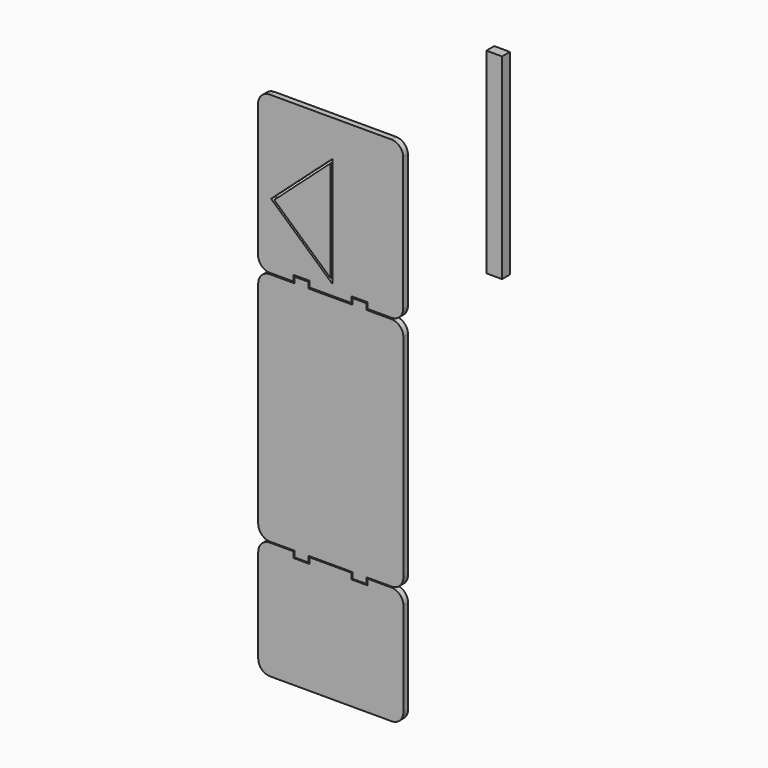
from build123d import *

# Parameters (mm, degrees)
F1_DEPTH = 15
F2_DEPTH = 15
F0_W     = 40
F0_H     = 500
F3_DEPTH = 25


# Not quite as in the source:
# - a feature names something its author has since deleted; it is built from what else it names


with BuildPart() as f1:
    # F0 (on Front) → F1 (new body)
    with BuildSketch(Plane.XZ):
        with BuildLine():
            Line((157.9930828999, 251.0488363948), (-152.0069171001, 251.0488363948))
            ThreePointArc((-152.0069171001, 251.0488363948), (-173.2201205357, 242.2620398304), (-182.0069171001, 221.0488363948))
            Line((-182.0069171001, 221.0488363948), (-182.0069171001, -118.9511636052))
            ThreePointArc((-182.0069171001, -118.9511636052), (-173.2201205357, -140.1643670408), (-152.0069171001, -148.9511636052))
            Line((-152.0069171001, -148.9511636052), (-91.4793238044, -148.9511636052))
            Line((-91.4793238044, -148.9511636052), (-91.4793238044, -133.9511636052))
            Line((-91.4793238044, -133.9511636052), (-51.4793238044, -133.9511636052))
            Line((-51.4793238044, -133.9511636052), (-51.4793238044, -148.9511636052))
            Line((-51.4793238044, -148.9511636052), (56.4180724323, -148.9511636052))
            Line((56.4180724323, -148.9511636052), (56.4180724323, -133.9511636052))
            Line((56.4180724323, -133.9511636052), (96.4180724323, -133.9511636052))
            Line((96.4180724323, -133.9511636052), (96.4180724323, -148.9511636052))
            Line((96.4180724323, -148.9511636052), (157.9930828999, -148.9511636052))
            ThreePointArc((157.9930828999, -148.9511636052), (179.2062863355, -140.1643670408), (187.9930828999, -118.9511636052))
            Line((187.9930828999, -118.9511636052), (187.9930828999, 221.0488363948))
            ThreePointArc((187.9930828999, 221.0488363948), (179.2062863355, 242.2620398304), (157.9930828999, 251.0488363948))
        make_face()
        Polygon((8.2889962941, 159.2487096786), (8.2889962941, -122.7074861526), (-148.9303992233, 18.270611763), align=None, mode=Mode.SUBTRACT)
    extrude(amount=F1_DEPTH)


with BuildPart() as f2:
    # F0 (on Front) → F2 (new body)
    with BuildSketch(Plane.XZ):
        with BuildLine():
            Line((-89.0557542443, -152.287649894), (-151.6510576755, -152.287649894))
            ThreePointArc((-151.6510576755, -152.287649894), (-172.8642611111, -161.0744464584), (-181.6510576755, -182.287649894))
            Line((-181.6510576755, -182.287649894), (-181.6510576755, -722.287649894))
            ThreePointArc((-181.6510576755, -722.287649894), (-172.8642611111, -743.5008533296), (-151.6510576755, -752.287649894))
            Line((-151.6510576755, -752.287649894), (-88.8991951942, -752.287649894))
            Line((-88.8991951942, -752.287649894), (-88.8991951942, -767.287649894))
            Line((-88.8991951942, -767.287649894), (-53.8991951942, -767.287649894))
            Line((-53.8991951942, -767.287649894), (-53.8991951942, -752.287649894))
            Line((-53.8991951942, -752.287649894), (59.3375265598, -752.287649894))
            Line((59.3375265598, -752.287649894), (59.3375265598, -767.287649894))
            Line((59.3375265598, -767.287649894), (94.3375265598, -767.287649894))
            Line((94.3375265598, -767.287649894), (94.3375265598, -752.287649894))
            Line((94.3375265598, -752.287649894), (158.3489423245, -752.287649894))
            ThreePointArc((158.3489423245, -752.287649894), (179.5621457601, -743.5008533296), (188.3489423245, -722.287649894))
            Line((188.3489423245, -722.287649894), (188.3489423245, -182.287649894))
            ThreePointArc((188.3489423245, -182.287649894), (179.5621457601, -161.0744464584), (158.3489423245, -152.287649894))
            Line((158.3489423245, -152.287649894), (94.114292264, -152.287649894))
            Line((94.114292264, -152.287649894), (94.114292264, -137.287649894))
            Line((94.114292264, -137.287649894), (59.114292264, -137.287649894))
            Line((59.114292264, -137.287649894), (59.114292264, -152.287649894))
            Line((59.114292264, -152.287649894), (-54.0557542443, -152.287649894))
            Line((-54.0557542443, -152.287649894), (-54.0557542443, -137.287649894))
            Line((-54.0557542443, -137.287649894), (-89.0557542443, -137.287649894))
            Line((-89.0557542443, -137.287649894), (-89.0557542443, -152.287649894))
        make_face()
    extrude(amount=F2_DEPTH)


with BuildPart() as f2b:
    # F0 (on Front) → F2, piece 2 (new body)
    with BuildSketch(Plane.XZ):
        with BuildLine():
            Line((-91.2640253641, -754.7138333321), (-151.6000044346, -754.7138333321))
            ThreePointArc((-151.6000044346, -754.7138333321), (-172.8132078702, -763.5006298965), (-181.6000044346, -784.7138333321))
            Line((-181.6000044346, -784.7138333321), (-181.6000044346, -1024.7138333321))
            ThreePointArc((-181.6000044346, -1024.7138333321), (-172.8132078702, -1045.9270367677), (-151.6000044346, -1054.7138333321))
            Line((-151.6000044346, -1054.7138333321), (-91.3764173724, -1054.7138333321))
            Line((-91.3764173724, -1054.7138333321), (56.5209788643, -1054.7138333321))
            Line((56.5209788643, -1054.7138333321), (158.3999955654, -1054.7138333321))
            ThreePointArc((158.3999955654, -1054.7138333321), (179.613199001, -1045.9270367677), (188.3999955654, -1024.7138333321))
            Line((188.3999955654, -1024.7138333321), (188.3999955654, -784.7138333321))
            ThreePointArc((188.3999955654, -784.7138333321), (179.613199001, -763.5006298965), (158.3999955654, -754.7138333321))
            Line((158.3999955654, -754.7138333321), (96.4699256234, -754.7138333321))
            Line((96.4699256234, -754.7138333321), (96.4699256234, -769.7138333321))
            Line((96.4699256234, -769.7138333321), (56.4699256234, -769.7138333321))
            Line((56.4699256234, -769.7138333321), (56.4699256234, -754.7138333321))
            Line((56.4699256234, -754.7138333321), (-51.2640253641, -754.7138333321))
            Line((-51.2640253641, -754.7138333321), (-51.2640253641, -769.7001099586))
            Line((-51.2640253641, -769.7001099586), (-91.2640253641, -769.7001099586))
            Line((-91.2640253641, -769.7001099586), (-91.2640253641, -754.7138333321))
        make_face()
    extrude(amount=F2_DEPTH)


with BuildPart() as f2c:
    # F0 (on Front) → F2, piece 3 (new body)
    with BuildSketch(Plane.XZ):
        Polygon((2.9930828999, -110.8454271421), (2.9930828999, 147.3866506681), (-140.9976921807, 18.270611763), align=None)
    extrude(amount=F2_DEPTH)


with BuildPart() as f3:
    # F0 (on Front) → F3 (new body)
    with BuildSketch(Plane.XZ):
        with Locations((428.1492424011, 285.9999984503)):
            Rectangle(F0_W, F0_H)
    extrude(amount=F3_DEPTH)


solid = Compound([f1.part, f2.part, f2b.part, f2c.part, f3.part])
